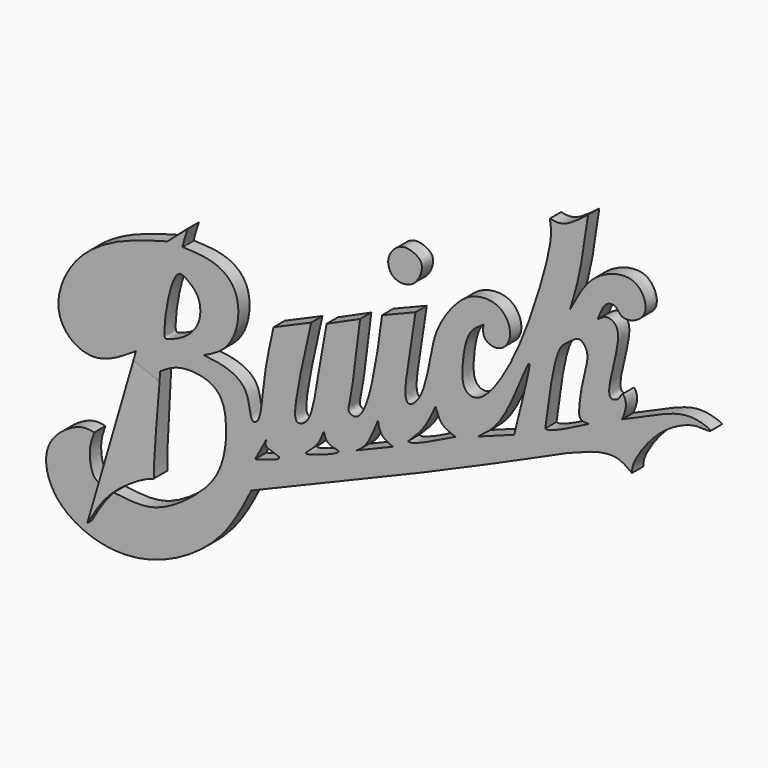
from build123d import *

# Parameters (mm, degrees)
F1_DEPTH    = 4.3
F2_DEPTH    = 6.2
F3_T4_DEPTH = 293.9876463293
F4_SCALE    = 0.9


# Not quite as in the source:
# - a fillet or chamfer that OpenCascade refuses, or shapes differently, is made with other operations: its cross-section is extruded or revolved along the edge and cut away or added


with BuildPart() as f1:
    # F0 (on Front) → F1 (new body)
    with BuildSketch(Plane.XZ):
        with BuildLine():
            add(Edge.make_bspline(
                [(-70.1490864158, -2.8128637932), (-67.6794399818, -3.8140723482), (-65.2097935478, -4.8152809031), (-62.7401471138, -5.8164894581)],
                knots=[0, 0, 0, 0, 7.994632494, 7.994632494, 7.994632494, 7.994632494], degree=3))
            add(Edge.make_bspline(
                [(-62.7401471138, -5.8164894581), (-60.8278243673, -4.5529948145), (-56.615185099, -1.7696498235), (-44.4004329285, -3.3433734498), (-41.8553850022, -13.8388396958), (-43.6777195032, -27.9087180168), (-53.3018071059, -37.1519235366), (-64.8678694935, -44.5384842868), (-72.9690368665, -43.4957610531), (-76.9006819092, -42.9933906453)],
                knots=[0, 0, 0, 0, 0.1148812894, 0.2530559346, 0.3846403677, 0.5431382402, 0.6981794491, 0.8534377949, 1, 1, 1, 1], degree=3))
            add(Edge.make_bspline(
                [(-76.9006819092, -42.9933906453), (-79.8017028101, -46.0033934894), (-81.683495051, -49.3382232429), (-83.565287292, -52.6730529964)],
                knots=[0.7765434948, 0.7765434948, 0.7765434948, 0.7765434948, 1, 1, 1, 1], degree=3))
            add(Edge.make_bspline(
                [(-83.565287292, -52.6730529964), (-82.606184594, -49.1086279829), (-81.6470818959, -45.5442029694), (-80.6879791979, -41.9797779558)],
                knots=[0, 0, 0, 0, 11.0736187835, 11.0736187835, 11.0736187835, 11.0736187835], degree=3))
            add(Edge.make_bspline(
                [(-82.8605219722, -28.7740267813), (-83.4573110239, -30.4133304366), (-84.7072892071, -33.846861596), (-83.5391188723, -41.1017063952), (-81.4762185611, -41.7370221996), (-80.6879791979, -41.9797779558)],
                knots=[0, 0, 0, 0, 0.3608364156, 0.7557739974, 1, 1, 1, 1], degree=3))
            add(Edge.make_bspline(
                [(-34.897275269, -28.7740267813), (-37.7432006712, -34.4433877201), (-43.6408278089, -46.1920361211), (-63.2695409394, -58.5280642117), (-81.5363494522, -59.2773706121), (-96.2681519356, -51.0216574299), (-99.469173215, -35.7342876811), (-87.6475116167, -27.8171011892), (-84.1740527929, -28.5114502245), (-82.8605219722, -28.7740267813)],
                knots=[0, 0, 0, 0, 0.1658665623, 0.3437262054, 0.5029253622, 0.6520629348, 0.7884391195, 0.9199956726, 1, 1, 1, 1], degree=3))
            add(Edge.make_bspline(
                [(81.2903046608, 13.6997839436), (79.9767842866, 14.6840672764), (77.0064789845, 16.9098584094), (67.6381533112, 15.9881848984), (37.2607489772, 1.0802909596), (-7.3505462149, -17.3769741251), (-34.897275269, -28.7740267813)],
                knots=[0, 0, 0, 0, 0.1123819244, 0.2541328116, 0.5394394792, 1, 1, 1, 1], degree=3))
            add(Edge.make_bspline(
                [(78.2686397433, 27.1499827504), (82.5266455861, 29.0767776297), (90.410268471, 32.6442044407), (99.021080305, 35.667565068), (107.1692572385, 32.5727605399), (102.4274805046, 32.7045653649), (98.9935172229, 32.8055844556), (89.0269849538, 28.1372091604), (81.4509169453, 17.1149279341), (81.3295752383, 14.5348052316), (81.2903046608, 13.6997839436)],
                knots=[0, 0, 0, 0, 0.1728670228, 0.3200602506, 0.4294811471, 0.5017305405, 0.592783119, 0.7475271149, 0.9182906171, 1, 1, 1, 1], degree=3))
            add(Edge.make_bspline(
                [(70.8170607686, 51.6188107431), (71.7338820187, 52.297243844), (73.5561527582, 53.6456951242), (77.6214023842, 51.8954783511), (76.6614302501, 44.0773524102), (74.1824763036, 35.6824330631), (74.3243185571, 30.9791988935), (77.5844603649, 32.0976289513), (78.3341105594, 34.8532393877), (80.0370083073, 31.507509392), (78.9302754772, 28.7803529098), (78.2686397433, 27.1499827504)],
                knots=[0, 0, 0, 0, 0.1007533928, 0.2002570944, 0.350867937, 0.52525071, 0.6275999793, 0.7149221617, 0.7914657765, 0.8753324287, 1, 1, 1, 1], degree=3))
            add(Edge.make_bspline(
                [(62.419552356, 51.6188107431), (64.5028613713, 55.5690836641), (68.3832141315, 62.9268267161), (78.1277127732, 66.6400154939), (84.0184541213, 65.0531446948), (86.5987000527, 58.2115282392), (82.0963739977, 54.3962541819), (77.750844678, 54.2679061091), (76.6671376765, 57.1769284813), (72.9503034634, 57.2414477799), (71.6147442281, 53.7212834594), (70.8170607686, 51.6188107431)],
                knots=[0, 0, 0, 0, 0.1682666237, 0.31341191, 0.4228693558, 0.5378215313, 0.644247026, 0.7349817332, 0.8101436339, 0.8866053419, 1, 1, 1, 1], degree=3))
            add(Edge.make_bspline(
                [(67.8872838616, 78.7345990539), (67.0703395147, 72.8350279025), (65.6004807537, 62.2204292758), (63.3979300863, 54.8796158229), (62.419552356, 51.6188107431)],
                knots=[0, 0, 0, 0, 0.5557978553, 1, 1, 1, 1], degree=3))
            add(Edge.make_bspline(
                [(56.2008656561, 73.9175602794), (57.5006474173, 73.6986409537), (60.723083907, 73.1558932059), (65.2101140439, 76.6499080887), (67.8872838616, 78.7345990539)],
                knots=[0, 0, 0, 0, 0.4033537248, 1, 1, 1, 1], degree=3))
            add(Edge.make_bspline(
                [(35.9471663833, 38.8244986534), (34.4207348249, 37.8822129269), (30.9127670378, 35.7166995393), (29.4244011351, 26.5088145334), (29.3825369561, 19.1336229359), (35.3360791212, 17.1531239243), (44.9500102271, 30.7105247133), (52.1459388369, 50.1961441537), (57.197735419, 68.5037211791), (56.4543716546, 72.5408100378), (56.2008656561, 73.9175602794)],
                knots=[0, 0, 0, 0, 0.0932514626, 0.2143057939, 0.3180882516, 0.3963059672, 0.548797467, 0.7409621764, 0.911661497, 1, 1, 1, 1], degree=3))
            add(Edge.make_bspline(
                [(15.2221424505, 35.4333035648), (14.2962906317, 29.5788530433), (12.7539503317, 19.8261531077), (11.8172196292, 12.2200794619), (12.9803912297, 9.3828923233), (17.3245217696, 12.5774439528), (19.7030576404, 23.8752350478), (21.0776809069, 33.003018055), (27.6585154052, 42.674517394), (33.9300748214, 46.5021863947), (42.0101452491, 45.9804918303), (45.3812812914, 38.2737349605), (41.1495295927, 32.9173670104), (35.583580464, 34.7337671572), (35.8298296015, 37.5043340278), (35.9471663833, 38.8244986534)],
                knots=[0, 0, 0, 0, 0.1187151001, 0.1977628378, 0.2373566712, 0.2941736185, 0.3933305327, 0.4848048072, 0.5821392994, 0.6603850178, 0.7376298439, 0.8148667305, 0.8832863981, 0.9443864105, 1, 1, 1, 1], degree=3))
            add(Edge.make_bspline(
                [(5.0098160282, 31.3154347241), (8.4139248356, 32.688057671), (11.8180336431, 34.0606806179), (15.2221424505, 35.4333035648)],
                knots=[0, 0, 0, 0, 11.0112876062, 11.0112876062, 11.0112876062, 11.0112876062], degree=3))
            add(Edge.make_bspline(
                [(-1.6982794041, 28.1115677208), (-2.7898745574, 18.8380968448), (-4.2880726003, 6.1103965857), (-5.7259697782, 1.8173110114), (-1.9754261674, 0.6425959488), (1.8500037622, 8.8234881719), (4.405550737, 26.4553132657), (4.858666161, 30.09973241), (5.0098160282, 31.3154347241)],
                knots=[0, 0, 0, 0, 0.2769987365, 0.3801766283, 0.4648379055, 0.6279510939, 0.8758922346, 1, 1, 1, 1], degree=3))
            add(Edge.make_bspline(
                [(-11.9106089696, 23.5060080886), (-8.5064991144, 25.0411946326), (-5.1023892593, 26.5763811767), (-1.6982794041, 28.1115677208)],
                knots=[0, 0, 0, 0, 11.2028056611, 11.2028056611, 11.2028056611, 11.2028056611], degree=3))
            add(Edge.make_bspline(
                [(-16.6162885725, 22.3045572639), (-18.750120908, 12.9409404674), (-21.7605886507, -0.2695006029), (-21.5544412388, -6.6479770515), (-16.649551873, -4.9527589187), (-14.7434542772, 7.801673593), (-12.9059936423, 17.9879327425), (-11.9106089696, 23.5060080886)],
                knots=[0, 0, 0, 0, 0.304191488, 0.4291614889, 0.5340617985, 0.7475930992, 1, 1, 1, 1], degree=3))
            add(Edge.make_bspline(
                [(-28.1301867217, 17.2985140234), (-24.292220672, 18.9671951036), (-20.4542546223, 20.6358761837), (-16.6162885725, 22.3045572639)],
                knots=[0, 0, 0, 0, 12.5550913781, 12.5550913781, 12.5550913781, 12.5550913781], degree=3))
            add(Edge.make_bspline(
                [(-49.4559295475, 2.8811094817), (-47.2939236559, 2.672434688), (-42.7986553461, 2.2385555804), (-35.2543285583, -1.4996990677), (-35.47288784, -10.652945479), (-31.8731531846, -9.5430956425), (-31.4459699658, 2.2464739125), (-29.3123790758, 11.9319368309), (-28.1301867217, 17.2985140234)],
                knots=[0, 0, 0, 0, 0.1553547726, 0.323015487, 0.4852026697, 0.5600337835, 0.7562209796, 1, 1, 1, 1], degree=3))
            add(Edge.make_bspline(
                [(-55.7635463774, 29.8265367746), (-52.1833246813, 29.6900823263), (-45.4606474512, 29.4338581897), (-38.6120542573, 23.6584983193), (-38.6088132025, 13.1405147035), (-43.0091662199, 5.8713902892), (-47.3678764738, 3.8496365881), (-49.4559295475, 2.8811094817)],
                knots=[0, 0, 0, 0, 0.2190367198, 0.4112910578, 0.6249998504, 0.8203550662, 1, 1, 1, 1], degree=3))
            add(Edge.make_bspline(
                [(-54.3299913406, 35.2330617607), (-55.177025441, 32.6359089816), (-56.1371174757, 29.6921010581), (-55.8029026444, 29.8123737733), (-55.7635463774, 29.8265367746)],
                knots=[0, 0, 0, 0, 0.8822426078, 1, 1, 1, 1], degree=3))
            add(Edge.make_bspline(
                [(-60.5374835432, 29.8265367746), (-57.8614650411, 32.2433532202), (-55.1854465391, 34.6601696657), (-54.3299913406, 35.2330617607)],
                knots=[0, 0, 0, 0, 0.8108834981, 0.8108834981, 0.8108834981, 0.8108834981], degree=3))
            add(Edge.make_bspline(
                [(-70.1490864158, -2.8128637932), (-74.1528595961, -5.3994151851), (-81.4058800303, -10.085072752), (-90.9697426626, -6.640358593), (-95.4133893146, 2.1996384917), (-89.880360052, 16.0891440287), (-76.838553151, 25.3540881328), (-66.0377905625, 28.3174431231), (-60.5374835432, 29.8265367746)],
                knots=[0, 0, 0, 0, 0.170115287, 0.3081717164, 0.4461347482, 0.6201708489, 0.8065713482, 1, 1, 1, 1], degree=3))
        make_face()
        with BuildLine():
            add(Edge.make_bspline(
                [(-30.2069429308, -13.4370410815), (-30.5015899123, -14.1900490749), (-31.2148604575, -16.0129030521), (-23.117153202, -17.0237014171), (-29.8560972157, -18.9040725105), (-33.7695628405, -19.9960488826)],
                knots=[0, 0, 0, 0, 0.2278626031, 0.5516013853, 1, 1, 1, 1], degree=3))
            add(Edge.make_bspline(
                [(-33.7695628405, -19.9960488826), (-32.5820228706, -17.8097129489), (-31.3944829007, -15.6233770152), (-30.2069429308, -13.4370410815)],
                knots=[0, 0, 0, 0, 7.4641036941, 7.4641036941, 7.4641036941, 7.4641036941], degree=3))
        make_face(mode=Mode.SUBTRACT)
        with BuildLine():
            add(Edge.make_bspline(
                [(-18.1181021035, -13.4370410815), (-18.8578846265, -13.3365862382), (-13.820171941, -10.3875690904), (-12.6943901401, -3.860686626), (-12.4008274549, -9.3180091725), (-4.0617156075, -9.0557999368), (-17.0274241508, -13.5851439081), (-18.1181021035, -13.4370410815)],
                knots=[0, 0, 0, 0, 0.19751706, 0.3899717884, 0.5420559599, 0.7087961719, 1, 1, 1, 1], degree=3))
        make_face(mode=Mode.SUBTRACT)
        with BuildLine():
            add(Edge.make_bspline(
                [(8.3146616817, -2.9534709174), (4.6025693106, -4.4860437823), (0.8904769396, -6.0186166471), (-2.8216154315, -7.551189512)],
                knots=[0, 0, 0, 0, 12.0480572797, 12.0480572797, 12.0480572797, 12.0480572797], degree=3))
            add(Edge.make_bspline(
                [(-2.8216154315, -7.551189512), (-1.8577206702, -6.9275366304), (0.5814811862, -5.349340205), (2.5719776924, -0.3481490044), (3.7758934777, 2.6767309755)],
                knots=[0, 0, 0, 0, 0.3951680992, 1, 1, 1, 1], degree=3))
            add(Edge.make_bspline(
                [(3.7758934777, 2.6767309755), (3.9900891245, 1.3851407294), (4.4267388312, -1.247837628), (7.0024491491, -2.3778027613), (8.3146616817, -2.9534709174)],
                knots=[0, 0, 0, 0, 0.4905434344, 1, 1, 1, 1], degree=3))
        make_face(mode=Mode.SUBTRACT)
        with BuildLine():
            add(Edge.make_bspline(
                [(27.4395365268, 5.9265033342), (21.960146218, 3.1968513184), (14.7835045267, -0.3783155078), (13.2829351579, -0.0723579283), (12.9280555993, 0)],
                knots=[0, 0, 0, 0, 0.7635033968, 1, 1, 1, 1], degree=3))
            add(Edge.make_bspline(
                [(12.9280555993, 0), (14.5476535324, 1.5372897566), (17.9354824085, 4.7529487311), (20.1651034402, 9.5832755547), (21.3288236409, 12.104398571)],
                knots=[0, 0, 0, 0, 0.478063678, 1, 1, 1, 1], degree=3))
            add(Edge.make_bspline(
                [(21.3288236409, 12.104398571), (21.8487797626, 10.5635238138), (22.885424041, 7.4914588175), (25.9246927414, 6.4470576894), (27.4395365268, 5.9265033342)],
                knots=[0, 0, 0, 0, 0.5015762228, 1, 1, 1, 1], degree=3))
        make_face(mode=Mode.SUBTRACT)
        with BuildLine():
            add(Edge.make_bspline(
                [(-57.5338602066, 21.816868335), (-60.0451297064, 19.2645545317), (-62.3312983819, 3.428148686), (-60.34771369, 3.5271181307), (-54.9213220148, 5.4914080791), (-50.0593893992, 10.9191410042), (-50.4724317803, 18.1533230027), (-53.8324515018, 21.0761868485), (-56.4401212956, 22.9284833648), (-57.5338602066, 21.816868335)],
                knots=[0, 0, 0, 0, 0.2545630088, 0.3109942824, 0.4504531489, 0.6110835029, 0.7620715158, 0.8891295944, 1, 1, 1, 1], degree=3))
        make_face(mode=Mode.SUBTRACT)
        with BuildLine():
            add(Edge.make_bspline(
                [(45.3290556379, 12.2851039218), (41.6448370124, 10.933236463), (37.9606183869, 9.5813690042), (34.2763997614, 8.2295015454)],
                knots=[0, 0, 0, 0, 11.7732371317, 11.7732371317, 11.7732371317, 11.7732371317], degree=3))
            add(Edge.make_bspline(
                [(34.2763997614, 8.2295015454), (36.3962750276, 9.7749742392), (41.3372865582, 13.3771665579), (46.8314538595, 26.2014088589), (49.6576692378, 33.2725375417), (50.4539955298, 32.0645010051), (45.7008872595, 14.204592511), (45.3570561162, 12.4506111294), (45.331786222, 12.2851255717)],
                knots=[0, 0, 0, 0, 0.1880111511, 0.4382169461, 0.5992840569, 0.6420942932, 0.9294942828, 0.9787091641, 0.9787091641, 0.9787091641, 0.9787091641], degree=3))
            Line((45.331786222, 12.2851255717), (45.3290556379, 12.2851039218))
        make_face(mode=Mode.SUBTRACT)
        with BuildLine():
            add(Edge.make_bspline(
                [(54.8220276833, 17.0376319438), (55.1502579899, 16.9694059262), (56.5417159872, 16.6801771869), (63.1851114891, 20.0693075224), (68.2613998652, 22.6589776576)],
                knots=[0, 0, 0, 0, 0.2358894823, 1, 1, 1, 1], degree=3))
            add(Edge.make_bspline(
                [(54.8220276833, 17.0376319438), (56.0803002222, 26.747503738), (57.8531220047, 40.4280631466), (62.0545253619, 42.4378149251), (65.3479192515, 45.5481703712), (68.476393604, 41.3693606581), (66.5603606578, 35.8591243904), (65.0268764772, 26.5762026108), (65.1632277749, 22.5147245711), (67.2672848067, 22.6126909565), (68.2613998652, 22.6589776576)],
                knots=[0, 0, 0, 0, 0.2482019493, 0.3496999326, 0.445097268, 0.5418123848, 0.6664494926, 0.8267652959, 0.9181508745, 1, 1, 1, 1], degree=3))
        make_face(mode=Mode.SUBTRACT)
    extrude(amount=F1_DEPTH)

    # F0 (on Front) → F2 (join)
    with BuildSketch(Plane.XZ):
        with BuildLine():
            add(Edge.make_bspline(
                [(-62.7401471138, -5.8164894581), (-63.4673103218, -18.4333390713), (-64.3173301951, -33.1818477855), (-63.7248461921, -34.7981828503), (-66.1739771984, -35.1209986174), (-73.0403729829, -39.1590021711), (-76.5973521619, -42.6786657835), (-76.9006819092, -42.9933906453)],
                knots=[0, 0, 0, 0, 0.3618024912, 0.4229302368, 0.5122688277, 0.7531789595, 0.7765434948, 0.7765434948, 0.7765434948, 0.7765434948], degree=3))
            add(Edge.make_bspline(
                [(-70.1490864158, -2.8128637932), (-67.6794399818, -3.8140723482), (-65.2097935478, -4.8152809031), (-62.7401471138, -5.8164894581)],
                knots=[0, 0, 0, 0, 7.994632494, 7.994632494, 7.994632494, 7.994632494], degree=3))
            add(Edge.make_bspline(
                [(-80.6879791979, -41.9797779558), (-77.1750149372, -28.9241399016), (-73.6620506765, -15.8685018474), (-70.1490864158, -2.8128637932)],
                knots=[11.0736187835, 11.0736187835, 11.0736187835, 11.0736187835, 51.6336412945, 51.6336412945, 51.6336412945, 51.6336412945], degree=3))
            add(Edge.make_bspline(
                [(-83.565287292, -52.6730529964), (-82.606184594, -49.1086279829), (-81.6470818959, -45.5442029694), (-80.6879791979, -41.9797779558)],
                knots=[0, 0, 0, 0, 11.0736187835, 11.0736187835, 11.0736187835, 11.0736187835], degree=3))
            add(Edge.make_bspline(
                [(-76.9006819092, -42.9933906453), (-79.8017028101, -46.0033934894), (-81.683495051, -49.3382232429), (-83.565287292, -52.6730529964)],
                knots=[0.7765434948, 0.7765434948, 0.7765434948, 0.7765434948, 1, 1, 1, 1], degree=3))
        make_face()
    extrude(amount=F2_DEPTH)

    # F3: chamfer of 2 x 55 on 1 edges, made by hand


with BuildPart() as f1b:
    # F0 (on Front) → F1, piece 2 (new body)
    with BuildSketch(Plane.XZ):
        with BuildLine():
            add(Edge.make_bspline(
                [(11.7103932425, 51.7724305391), (10.0736133718, 51.5975380318), (7.5248195558, 49.4942239878), (6.4084223816, 45.7366975982), (8.5244944769, 41.5737205139), (14.8979078285, 41.7732742545), (17.4696238521, 47.1265236371), (17.008621496, 50.4707029954), (13.4238510053, 51.9555162), (11.7103932425, 51.7724305391)],
                knots=[0, 0, 0, 0, 0.1467786644, 0.2780625807, 0.4133530903, 0.5707257543, 0.7290306174, 0.8463452255, 1, 1, 1, 1], degree=3))
        make_face()
    extrude(amount=F1_DEPTH)


with BuildPart() as f3_tool2:
    # F3_s3 → F3_t4 (new body)
    with BuildSketch(Plane(origin=(-191.7883128853, 0, 77.7520607639), x_dir=(0, 1, 0), z_dir=(0.9267391975, 0, -0.3757052832))):
        Polygon((-4.2, -28.962173509), (-6.2, -83.962173509), (-6.2, -28.962173509), align=None)
    extrude(amount=F3_T4_DEPTH)

    split(bisect_by=Plane.XZ.offset(4.3), keep=Keep.TOP)


with BuildPart() as f1_1:
    add(f1.part)

    # F3_t1: cut F3_tool2
    add(f3_tool2.part, mode=Mode.SUBTRACT)


with BuildPart() as f1_2:
    # F4: moved
    add(f1_1.part.scale(F4_SCALE))


with BuildPart() as f1b_1:
    # F4: moved
    add(f1b.part.scale(F4_SCALE))


solid = Compound([f1_2.part, f1b_1.part])
